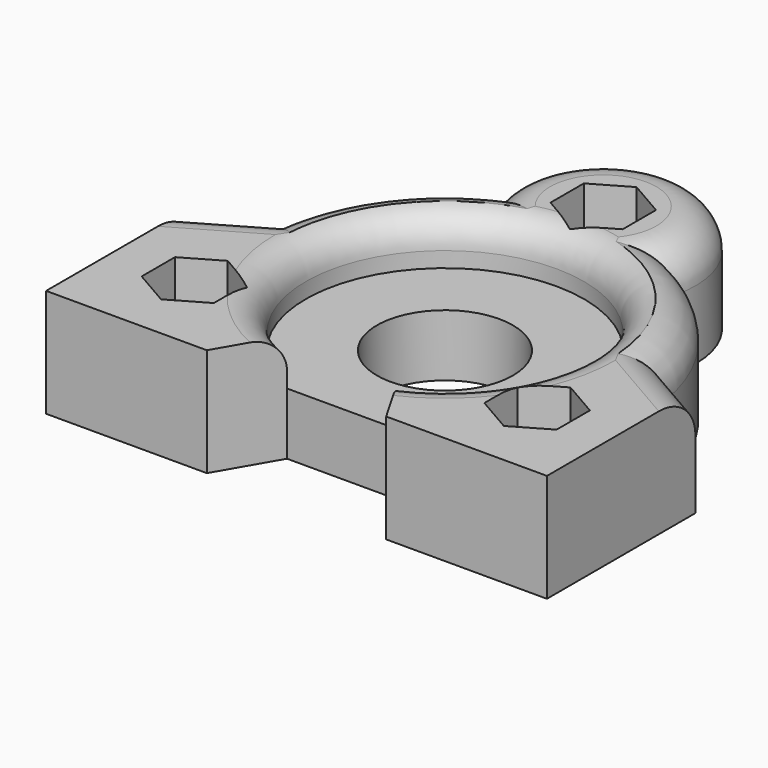
from build123d import *

# Parameters (mm, degrees)
F0_R          = 2.125
F0_R_2        = 5.25
F1_DEPTH      = 5
F3_DEPTH      = 15
F4_R          = 2.125
F5_DEPTH      = 25
F6_W          = 50
F6_H          = 15
F6_R          = 2.125
F7_DEPTH      = 5
F8_R          = 7.5
F9_SIZE       = 7.5
F10_R         = 11.25
F11_DEPTH     = 3.75
F12_T1_DEPTH  = 10
F12_T6_DEPTH  = 4
F12_S7_R      = 25
F12_T8_DEPTH  = 4
F12_T12_DEPTH = 4
F12_S13_R     = 25
F12_T14_DEPTH = 4
F13_R         = 4.99999
F14_R         = 1.99999
F15_R         = 5.5
F16_DEPTH     = 25
F18_DEPTH     = 17.5
F19_R         = 3.2
F20_T2_ANGLE  = 359.64


# Not quite as in the source:
# - a fillet or chamfer that OpenCascade refuses, or shapes differently, is made with other operations: its cross-section is extruded or revolved along the edge and cut away or added
# - a fillet or chamfer is up to 0.001 mm smaller than in the source, because OpenCascade refuses the exact size


with BuildPart() as f1:
    # F0 (on Top) → F1 (new body)
    with BuildSketch(Plane.XY):
        with BuildLine():
            Line((25, -27.1), (25, -22.1))
            Line((25, -22.1), (25, 0))
            ThreePointArc((25, 0), (0, 25), (-25, 0))
            Line((-25, 0), (-25, -22.1))
            Line((-25, -22.1), (-25, -27.1))
            Line((-25, -27.1), (25, -27.1))
        make_face()
        with Locations((-13.856406, -8)):
            Circle(F0_R, mode=Mode.SUBTRACT)
        with Locations((13.856406, -8)):
            Circle(F0_R, mode=Mode.SUBTRACT)
        Circle(F0_R_2, mode=Mode.SUBTRACT)
        with Locations((0, 16)):
            Circle(F0_R, mode=Mode.SUBTRACT)
    extrude(amount=F1_DEPTH)

    # F2 (on face) → F3 (join)
    with BuildSketch(Plane.XY.offset(5)):
        Polygon((-25, -27.1), (25, -27.1), (25, -22.1), (25, 0), (21, 0), (21, -22.1), (5, -22.1), (5, -14.1), (0, -14.1), (-5, -14.1), (-5, -22.1), (-21, -22.1), (-21, 0), (-25, 0), (-25, -22.1), align=None)
    extrude(amount=F3_DEPTH)

    # F4 (on face) → F5 (cut)
    with BuildSketch(Plane.XZ.offset(27.1)):
        with Locations((-11.725, 12.5)):
            Circle(F4_R)
        with Locations((11.725, 12.5)):
            Circle(F4_R)
    extrude(amount=-F5_DEPTH, mode=Mode.SUBTRACT)

    # F6 (on Top) → F7 (join)
    with BuildSketch(Plane.XY):
        with Locations((0, -34.6)):
            Rectangle(F6_W, F6_H)
        with Locations((-17.5, -34.6)):
            Circle(F6_R, mode=Mode.SUBTRACT)
        with Locations((17.5, -34.6)):
            Circle(F6_R, mode=Mode.SUBTRACT)
    extrude(amount=F7_DEPTH)

    # F8
    f8_edges = [f1.edges().sort_by_distance(p)[0] for p in [
        (-25, -42.1, 2.5),
        (25, -42.1, 2.5),
    ]]
    fillet(f8_edges, radius=F8_R)

    # F9
    f9_edges = [f1.edges().sort_by_distance(p)[0] for p in [
        (0, -14.1, 20),
        (-23, 0, 20),
        (23, 0, 20),
    ]]
    chamfer(f9_edges, length=F9_SIZE)

    # F10 (on face) → F11 (join)
    with BuildSketch(Plane.XY.offset(5)):
        with BuildLine():
            Line((25, -22.1), (25, 0))
            ThreePointArc((25, 0), (0, 25), (-25, 0))
            Line((-25, 0), (-25, -22.1))
            Line((-25, -22.1), (25, -22.1))
        make_face()
        Polygon((-16.773906, -9.684419), (-16.773906, -6.315581), (-13.856406, -4.631161), (-10.938906, -6.315581), (-10.938906, -9.684419), (-13.856406, -11.368839), align=None, mode=Mode.SUBTRACT)
        Circle(F10_R, mode=Mode.SUBTRACT)
        Polygon((13.856406, -4.631161), (16.773906, -6.315581), (16.773906, -9.684419), (13.856406, -11.368839), (10.938906, -9.684419), (10.938906, -6.315581), align=None, mode=Mode.SUBTRACT)
        Polygon((0, 19.368839), (2.9175, 17.684419), (2.9175, 14.315581), (0, 12.631161), (-2.9175, 14.315581), (-2.9175, 17.684419), align=None, mode=Mode.SUBTRACT)
    extrude(amount=F11_DEPTH)

    # F12: chamfer of 2.5 on 3 edges, made by hand

    # F12_s2 → F12_t1 (join)
    with BuildSketch(Plane.YZ.offset(-5)):
        with BuildLine():
            Line((-14.170711, 11.320711), (-11.529289, 8.679289))
            Line((-11.529289, 8.679289), (-11.529289, 8.629289))
            ThreePointArc((-11.529289, 8.629289), (-12.814645, 8.7), (-14.1, 8.7))
            Line((-14.1, 8.7), (-14.15, 8.75))
            ThreePointArc((-14.15, 8.75), (-14.15, 10.035355), (-14.220711, 11.320711))
            Line((-14.220711, 11.320711), (-14.170711, 11.320711))
        make_face()
    extrude(amount=F12_T1_DEPTH)


with BuildPart() as f12_tool4:
    # F12_s5 → F12_t6 (new body)
    with BuildSketch(Plane.YZ.offset(-21)):
        with BuildLine():
            Line((-0.070711, 11.320711), (2.570711, 8.679289))
            Line((2.570711, 8.679289), (2.570711, 8.629289))
            ThreePointArc((2.570711, 8.629289), (1.285355, 8.7), (0, 8.7))
            Line((0, 8.7), (-0.05, 8.75))
            ThreePointArc((-0.05, 8.75), (-0.05, 10.035355), (-0.120711, 11.320711))
            Line((-0.120711, 11.320711), (-0.070711, 11.320711))
        make_face()
    extrude(amount=-F12_T6_DEPTH)

    # F12_s7 → F12_t8 (intersect, symmetric)
    with BuildSketch(Plane.XY.offset(10)):
        Circle(F12_S7_R)
    extrude(amount=F12_T8_DEPTH, both=True, mode=Mode.INTERSECT)


with BuildPart() as f1_1:
    add(f1.part)

    # F12_t3: union F12_tool4
    add(f12_tool4.part)


with BuildPart() as f12_tool10:
    # F12_s11 → F12_t12 (new body)
    with BuildSketch(Plane.YZ.offset(25)):
        with BuildLine():
            Line((2.570711, 8.679289), (-0.070711, 11.320711))
            Line((-0.070711, 11.320711), (-0.120711, 11.320711))
            ThreePointArc((-0.120711, 11.320711), (-0.05, 10.035355), (-0.05, 8.75))
            Line((-0.05, 8.75), (0, 8.7))
            ThreePointArc((0, 8.7), (1.285355, 8.7), (2.570711, 8.629289))
            Line((2.570711, 8.629289), (2.570711, 8.679289))
        make_face()
    extrude(amount=-F12_T12_DEPTH)

    # F12_s13 → F12_t14 (intersect, symmetric)
    with BuildSketch(Plane.XY.offset(10)):
        Circle(F12_S13_R)
    extrude(amount=F12_T14_DEPTH, both=True, mode=Mode.INTERSECT)


with BuildPart() as f1_2:
    add(f1_1.part)

    # F12_t9: union F12_tool10
    add(f12_tool10.part)

    # F13 (radius 5 in the source; OpenCascade refuses exactly that, so slightly less here)
    f13_edges = [f1_2.edges().sort_by_distance(p)[0] for p in [
        (5, -17.85, 16.25),
        (-5, -17.85, 16.25),
    ]]
    fillet(f13_edges, radius=F13_R)

    # F14 (radius 2 in the source; OpenCascade refuses exactly that, so slightly less here)
    f14_edges = [f1_2.edges().sort_by_distance(p)[0] for p in [
        (21, -14.8, 20),
        (25, -17.3, 20),
        (-21, -14.8, 20),
        (-25, -17.3, 20),
    ]]
    fillet(f14_edges, radius=F14_R)

    # F15 (on face) → F16 (cut)
    with BuildSketch(Plane.XY.offset(5)):
        Circle(F15_R)
    extrude(amount=-F16_DEPTH, mode=Mode.SUBTRACT)

    # F17 (on face) → F18 (cut, symmetric)
    with BuildSketch(Plane.XY.offset(5)):
        with BuildLine():
            ThreePointArc((0, 25), (-17.67767, 17.67767), (-25, 0))
            Line((-25, 0), (-25, -42.1))
            Line((-25, -42.1), (0, -42.1))
            Line((0, -42.1), (25, -42.1))
            Line((25, -42.1), (25, 0))
            ThreePointArc((25, 0), (17.67767, 17.67767), (0, 25))
        make_face()
        with BuildLine():
            ThreePointArc((-7.291097, 14.242188), (0, 23.5), (7.291097, 14.242188))
            ThreePointArc((7.291097, 14.242188), (12.932085, 9.421315), (15.791586, 2.574067))
            Line((15.791586, 2.574067), (20.25, 0))
            Line((20.25, 0), (20.25, -15))
            Line((20.25, -15), (7.25, -15))
            Line((7.25, -15), (4.534064, -10.295861))
            Line((4.534064, -10.295861), (-4.534064, -10.295861))
            Line((-4.534064, -10.295861), (-7.25, -15))
            Line((-7.25, -15), (-20.25, -15))
            Line((-20.25, -15), (-20.25, 0))
            Line((-20.25, 0), (-15.791586, 2.574067))
            ThreePointArc((-15.791586, 2.574067), (-12.932085, 9.421315), (-7.291097, 14.242188))
        make_face(mode=Mode.SUBTRACT)
    extrude(amount=F18_DEPTH, both=True, mode=Mode.SUBTRACT)

    # F19
    f19_edges = [f1_2.edges().sort_by_distance(p)[0] for p in [
        (0, 23.5, 8.75),
        (-12.932085, 9.421315, 8.75),
        (12.932085, 9.421315, 8.75),
        (-18.020793, 1.287033, 8.75),
        (18.020793, 1.287033, 8.75),
    ]]
    fillet(f19_edges, radius=F19_R)

    # F20: fillet of radius 2.5 on 1 edges, made by hand

    # F20_s1 → F20_t2 (revolve, cut)
    with BuildSketch(Plane(origin=(0, 0, 0), x_dir=(0, 0, 1), z_dir=(0.999995, -0.003142, 0))):
        with BuildLine():
            ThreePointArc((8.75, 13.75), (8.017767, 11.982233), (6.25, 11.25))
            Line((6.25, 11.25), (8.75, 11.25))
            Line((8.75, 11.25), (8.75, 13.75))
        make_face()
    revolve(axis=Axis((0, 0, 8.75), (0, 0, -1)), revolution_arc=F20_T2_ANGLE, mode=Mode.SUBTRACT)


solid = f1_2.part
